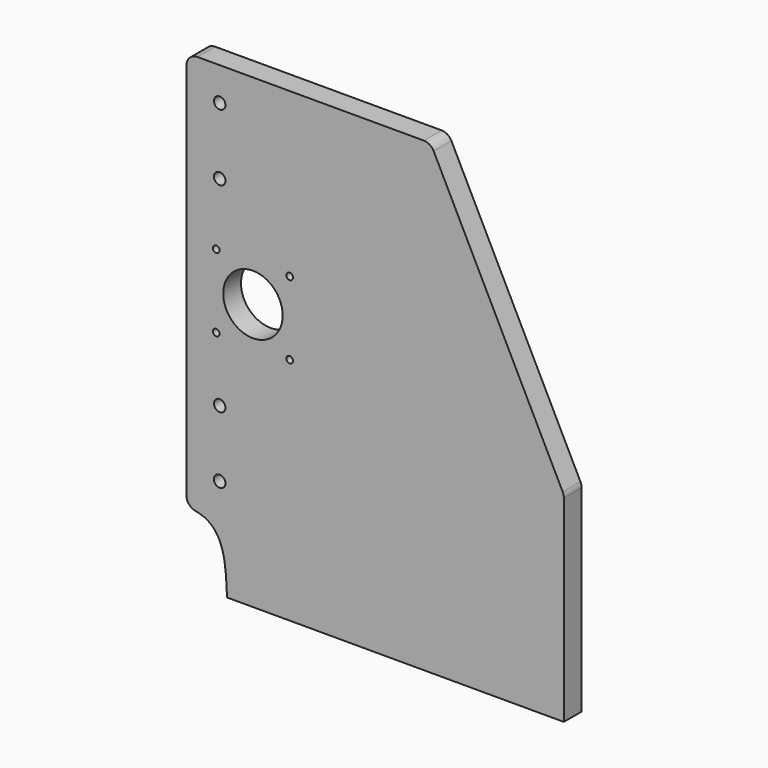
from build123d import *

# Parameters (mm, degrees)
F0_R     = 3.302
F0_W     = 52
F0_H     = 52
F0_R_2   = 1.9128263044
F0_R_3   = 17
F1_DEPTH = 12.7
F2_DEPTH = 25.4
F3_R     = 6.35


with BuildPart() as f1:
    # F0 (on Front) → F1 (new body)
    with BuildSketch(Plane.XZ):
        with BuildLine():
            Line((108.4265169831, 0.0004552842), (32.2265169831, 152.4004552842))
            Line((32.2265169831, 152.4004552842), (-107.4734830169, 152.4004552842))
            Line((-107.4734830169, 152.4004552842), (-107.4734830169, -76.1995447158))
            add(Edge.make_bspline(
                [(-84.2229677556, -114.2995447158), (-85.0358593396, -95.7832909802), (-85.4194185281, -76.1871889735), (-107.4734830169, -76.1995447158)],
                knots=[0, 0, 0, 0, 44.6340280494, 44.6340280494, 44.6340280494, 44.6340280494], degree=3))
            Line((-84.2229677556, -114.2995447158), (108.4265169831, -114.2995447158))
            Line((108.4265169831, -114.2995447158), (108.4265169831, 0.0004552842))
        make_face()
        with Locations((-88.4234830169, -57.1371889735)):
            Circle(F0_R, mode=Mode.SUBTRACT)
        with Locations((-88.4234830169, -19.0371889735)):
            Circle(F0_R, mode=Mode.SUBTRACT)
        with Locations((-69.4084768891, 38.0714893565)):
            Rectangle(F0_W, F0_H, mode=Mode.SUBTRACT)
        with Locations((-88.4234830169, 95.2504552842)):
            Circle(F0_R, mode=Mode.SUBTRACT)
        with Locations((-88.4234830169, 133.3504552842)):
            Circle(F0_R, mode=Mode.SUBTRACT)
        with Locations((-69.4084768891, 38.0714893565)):
            Rectangle(F0_W, F0_H)
        with Locations((-90.4046768891, 17.0752893565)):
            Circle(F0_R_2, mode=Mode.SUBTRACT)
        with Locations((-48.4122768891, 17.0752893565)):
            Circle(F0_R_2, mode=Mode.SUBTRACT)
        with Locations((-69.4084763527, 38.0714898929)):
            Circle(F0_R_3, mode=Mode.SUBTRACT)
        with Locations((-90.4046768891, 59.0676893565)):
            Circle(F0_R_2, mode=Mode.SUBTRACT)
        with Locations((-48.4122768891, 59.0676893565)):
            Circle(F0_R_2, mode=Mode.SUBTRACT)
    extrude(amount=F1_DEPTH)

    # F0 (on Front) → F2 (cut)
    with BuildSketch(Plane.XZ):
        with BuildLine():
            Line((108.4265169831, 0.0004552842), (32.2265169831, 152.4004552842))
            Line((32.2265169831, 152.4004552842), (-107.4734830169, 152.4004552842))
            Line((-107.4734830169, 152.4004552842), (-107.4734830169, -76.1995447158))
            add(Edge.make_bspline(
                [(-84.2229677556, -114.2995447158), (-85.0358593396, -95.7832909802), (-85.4194185281, -76.1871889735), (-107.4734830169, -76.1995447158)],
                knots=[0, 0, 0, 0, 44.6340280494, 44.6340280494, 44.6340280494, 44.6340280494], degree=3))
            Line((-84.2229677556, -114.2995447158), (108.4265169831, -114.2995447158))
            Line((108.4265169831, -114.2995447158), (108.4265169831, 0.0004552842))
        make_face()
        with Locations((-88.4234830169, -57.1371889735)):
            Circle(F0_R, mode=Mode.SUBTRACT)
        with Locations((-88.4234830169, -19.0371889735)):
            Circle(F0_R, mode=Mode.SUBTRACT)
        with Locations((-69.4084768891, 38.0714893565)):
            Rectangle(F0_W, F0_H, mode=Mode.SUBTRACT)
        with Locations((-88.4234830169, 95.2504552842)):
            Circle(F0_R, mode=Mode.SUBTRACT)
        with Locations((-88.4234830169, 133.3504552842)):
            Circle(F0_R, mode=Mode.SUBTRACT)
    extrude(amount=-F2_DEPTH, mode=Mode.SUBTRACT)

    # F3
    f3_edges = [f1.edges().sort_by_distance(p)[0] for p in [
        (-107.473483, -6.35, 152.400455),
        (-107.473483, -6.35, -76.199545),
        (108.426517, -6.35, 0.000455),
        (32.226517, -6.35, 152.400455),
    ]]
    fillet(f3_edges, radius=F3_R)


solid = f1.part
